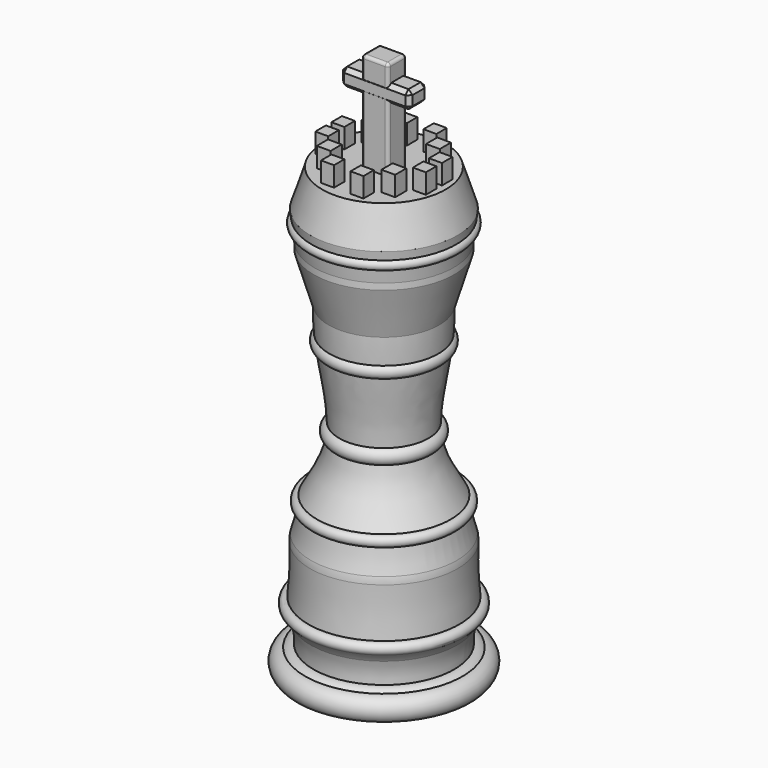
from build123d import *

# Parameters (mm, degrees)
F2_R         = 5.08
F3_W         = 3.3200064208
F3_H         = 3.3200057223
F3_W_2       = 3.5232715309
F3_H_2       = 3.5910271108
F3_W_3       = 3.3200057223
F3_H_3       = 3.3877615933
F4_DEPTH     = 5.08
F6_DEPTH     = 25.4
F7_W         = 5.9285820462
F7_H         = 4.5396015048
F8_DEPTH     = 8.89
F9_T1_DEPTH  = 1.2904933217
F9_T3_DEPTH  = 1.2904933217
F9_T5_DEPTH  = 1.2904933217
F9_T7_DEPTH  = 1.2904933217
F9_T9_DEPTH  = 1.2904933217
F9_T11_DEPTH = 1.2904933217
F9_T13_DEPTH = 1.2904933217
F9_T15_DEPTH = 1.2904933217
F9_T17_DEPTH = 9.7652613363
F9_T19_DEPTH = 11.1542418777
F9_T24_DEPTH = 23.0056598315
F9_T29_DEPTH = 23.0056598315
F9_T34_DEPTH = 23.0056598315
F9_T39_DEPTH = 23.0056598315
F9_T44_DEPTH = 23.0056598315
F9_T49_DEPTH = 23.0056598315
F9_T54_DEPTH = 23.0056598315
F9_T59_DEPTH = 23.0056598315
F9_T64_DEPTH = 23.0056598315
F9_T69_DEPTH = 23.0056598315
F9_T74_DEPTH = 23.0056598315
F9_T79_DEPTH = 23.0056598315
F10_R        = 0.762


# Not quite as in the source:
# - a fillet or chamfer that OpenCascade refuses, or shapes differently, is made with other operations: its cross-section is extruded or revolved along the edge and cut away or added


with BuildPart() as f1:
    # F0 (on Front) → F1 (revolve)
    with BuildSketch(Plane.XZ):
        with BuildLine():
            Line((0, -44.1694706678), (0, -37.9232913257))
            Line((0, -37.9232913257), (0, 63.8088807464))
            Line((0, 63.8088807464), (0, 69.7572231293))
            Line((0, 69.7572231293), (-15.8390831202, 69.7572231293))
            Line((-15.8390831202, 69.7572231293), (-18.8497721448, 60.3641234338))
            Line((-18.8497721448, 60.3641234338), (-18.5980623237, 58.2668431447))
            Line((-18.5980623237, 58.2668431447), (-18.3204592247, 55.9538165611))
            Line((-18.3204592247, 55.9538165611), (-17.942056863, 52.8009168813))
            Line((-17.942056863, 52.8009168813), (-17.9805713706, 51.2068634213))
            Line((-17.9805713706, 51.2068634213), (-14.2099214718, 38.6048460963))
            add(Edge.make_bspline(
                [(-13.9907028054, 32.0658987042), (-14.0967334303, 33.1756452858), (-14.2488688656, 35.3679737242), (-14.2418096298, 37.5414304271), (-14.2099214718, 38.6048460963)],
                knots=[0.6441859046, 0.6441859046, 0.6441859046, 0.6441859046, 0.6711541365, 0.6974927035, 0.6974927035, 0.6974927035, 0.6974927035], degree=3))
            add(Edge.make_bspline(
                [(-13.6247694985, 28.9412781618), (-13.765929725, 29.9810613532), (-13.8911317436, 31.0237597427), (-13.9907028054, 32.0658987042)],
                knots=[0.6188606226, 0.6188606226, 0.6188606226, 0.6188606226, 0.6441859046, 0.6441859046, 0.6441859046, 0.6441859046], degree=3))
            add(Edge.make_bspline(
                [(-11.4472950696, 12.1344692159), (-11.504994338, 17.2174563495), (-12.8225699529, 23.0322935701), (-13.6247694985, 28.9412781618)],
                knots=[0.4749395602, 0.4749395602, 0.4749395602, 0.4749395602, 0.6188606226, 0.6188606226, 0.6188606226, 0.6188606226], degree=3))
            add(Edge.make_bspline(
                [(-11.675667949, 8.4173418581), (-11.4991159546, 9.6023314431), (-11.4326559718, 10.8448454905), (-11.4472950696, 12.1344692159)],
                knots=[0.4384248078, 0.4384248078, 0.4384248078, 0.4384248078, 0.4749395602, 0.4749395602, 0.4749395602, 0.4749395602], degree=3))
            add(Edge.make_bspline(
                [(-17.1511071188, -4.3389676859), (-14.8148615903, -0.088300858), (-12.3768989208, 3.7107884096), (-11.675667949, 8.4173418581)],
                knots=[0.2933951502, 0.2933951502, 0.2933951502, 0.2933951502, 0.4384248078, 0.4384248078, 0.4384248078, 0.4384248078], degree=3))
            ThreePointArc((-17.1511071188, -4.3389676859), (-17.2505902332, -5.7148781332), (-17.4047115493, -7.0857439431))
            ThreePointArc((-17.4047115493, -7.0857439431), (-18.0433576285, -10.5447425672), (-19.0290799315, -13.9212632375))
            ThreePointArc((-19.0290799315, -13.9212632375), (-18.9285766864, -20.6231104547), (-19.3779931732, -27.3106273217))
            ThreePointArc((-19.3779931732, -27.3106273217), (-19.5478697821, -28.7552418846), (-19.7434488019, -30.1966017093))
            ThreePointArc((-19.7434488019, -30.1966017093), (-18.3122766997, -33.9317340327), (-18.0535539985, -37.9232913257))
            ThreePointArc((-18.0535539985, -37.9232913257), (-19.2128837803, -38.1464424542), (-20.2065406059, -38.7840066329))
            ThreePointArc((-20.2065406059, -38.7840066329), (-20.9534925411, -42.2057107785), (-18.0535539985, -44.1694706678))
            Line((-18.0535539985, -44.1694706678), (0, -44.1694706678))
        make_face()
        with BuildLine():
            Line((-22.0736673223, -44.1694706678), (-18.0535539985, -44.1694706678))
            ThreePointArc((-18.0535539985, -44.1694706678), (-20.9534925411, -42.2057107785), (-20.2065406059, -38.7840066329))
            ThreePointArc((-20.2065406059, -38.7840066329), (-22.963549203, -40.8445548127), (-22.0736673223, -44.1694706678))
        make_face()
        with BuildLine():
            Line((-18.3204592247, 55.9538165611), (-18.5980623237, 58.2668431447))
            ThreePointArc((-18.5980623237, 58.2668431447), (-19.40314177, 56.9970478477), (-18.3204592247, 55.9538165611))
        make_face()
        with BuildLine():
            ThreePointArc((-19.3779931732, -27.3106273217), (-21.0588794116, -28.5639002786), (-19.7434488019, -30.1966017093))
            ThreePointArc((-19.7434488019, -30.1966017093), (-19.5478697821, -28.7552418846), (-19.3779931732, -27.3106273217))
        make_face()
        with BuildLine():
            ThreePointArc((-18.3504191868, -6.6034462951), (-17.925820634, -6.9392158865), (-17.4047115493, -7.0857439431))
            ThreePointArc((-17.4047115493, -7.0857439431), (-17.2505902332, -5.7148781332), (-17.1511071188, -4.3389676859))
            add(Edge.make_bspline(
                [(-18.3504191868, -6.6034462951), (-17.9601567988, -5.8302207751), (-17.55716838, -5.0777732233), (-17.1511071188, -4.3389676859)],
                knots=[0.2681876432, 0.2681876432, 0.2681876432, 0.2681876432, 0.2933951502, 0.2933951502, 0.2933951502, 0.2933951502], degree=3))
        make_face()
        with BuildLine():
            add(Edge.make_bspline(
                [(-18.3504191868, -6.6034462951), (-17.9601567988, -5.8302207751), (-17.55716838, -5.0777732233), (-17.1511071188, -4.3389676859)],
                knots=[0.2681876432, 0.2681876432, 0.2681876432, 0.2681876432, 0.2933951502, 0.2933951502, 0.2933951502, 0.2933951502], degree=3))
            ThreePointArc((-17.1511071188, -4.3389676859), (-18.5181267124, -5.0647962725), (-18.3504191868, -6.6034462951))
        make_face()
        with BuildLine():
            add(Edge.make_bspline(
                [(-13.6247694985, 28.9412781618), (-13.765929725, 29.9810613532), (-13.8911317436, 31.0237597427), (-13.9907028054, 32.0658987042)],
                knots=[0.6188606226, 0.6188606226, 0.6188606226, 0.6188606226, 0.6441859046, 0.6441859046, 0.6441859046, 0.6441859046], degree=3))
            ThreePointArc((-13.9907028054, 32.0658987042), (-14.8106984904, 30.3861286262), (-13.6247694985, 28.9412781618))
        make_face()
        with BuildLine():
            ThreePointArc((-11.4472950696, 12.1344692159), (-12.8496274606, 10.355046651), (-11.675667949, 8.4173418581))
            add(Edge.make_bspline(
                [(-11.675667949, 8.4173418581), (-11.4991159546, 9.6023314431), (-11.4326559718, 10.8448454905), (-11.4472950696, 12.1344692159)],
                knots=[0.4384248078, 0.4384248078, 0.4384248078, 0.4384248078, 0.4749395602, 0.4749395602, 0.4749395602, 0.4749395602], degree=3))
        make_face()
    revolve(axis=Axis((0, 0, 12.9427947103), (0, 0, 1)))

    # F2
    f2_edges = [f1.edges().sort_by_distance(p)[0] for p in [
        (19.743449, 0, -30.196602),
        (19.02908, 0, -13.921263),
    ]]
    fillet(f2_edges, radius=F2_R)

    # F3 (on face) → F4 (join)
    with BuildSketch(Plane.XY.offset(69.7572231293)):
        with Locations((-3.7773378426, 11.6962320171)):
            Rectangle(F3_W, F3_H)
        with Locations((3.7773378426, 11.6962320171)):
            Rectangle(F3_W, F3_H)
        with Locations((-3.7773378426, -11.6962320171)):
            Rectangle(F3_W, F3_H)
        with Locations((3.7773378426, -11.6962320171)):
            Rectangle(F3_W, F3_H)
        with Locations((-8.2830600441, 7.1566319093)):
            Rectangle(F3_W_2, F3_H_2)
        with Locations((-8.2830600441, -7.1566319093)):
            Rectangle(F3_W_2, F3_H_2)
        with Locations((8.2830600441, 7.1566319093)):
            Rectangle(F3_W_2, F3_H_2)
        with Locations((8.2830600441, -7.1566319093)):
            Rectangle(F3_W_2, F3_H_2)
        with Locations((-12.5177619047, 2.583153866)):
            Rectangle(F3_W_3, F3_H_3)
        with Locations((-12.5177619047, -2.583153866)):
            Rectangle(F3_W_3, F3_H_3)
        with Locations((12.5177619047, 2.583153866)):
            Rectangle(F3_W_3, F3_H_3)
        with Locations((12.5177619047, -2.583153866)):
            Rectangle(F3_W_3, F3_H_3)
    extrude(amount=F4_DEPTH)

    # F5 (on face) → F6 (join)
    with BuildSketch(Plane.XY.offset(69.7572231293)):
        Polygon((3.4440401942, 2.9264579061), (0, 2.9264579061), (-3.4440401942, 2.9264579061), (-3.4440401942, 0), (-3.4440401942, -2.9264579061), (0, -2.9264579061), (3.4440401942, -2.9264579061), (3.4440401942, 0), align=None)
    extrude(amount=F6_DEPTH)

    # F7 (on Right) → F8 (join, symmetric)
    with BuildSketch(Plane.YZ):
        with Locations((0.0055725686, 88.3572287858)):
            Rectangle(F7_W, F7_H)
    extrude(amount=F8_DEPTH, both=True)

    # F9: chamfer of 1.016 on 12 edges, made by hand

    # F9_s2 → F9_t1 (cut)
    with BuildSketch(Plane(origin=(-33.4812493309, -33.4812493309, 33.4812493309), x_dir=(0.7071067812, -0.7071067812, 0), z_dir=(-0.5773502692, -0.5773502692, 0.5773502692))):
        Polygon((-4.9124698917, 68.7446604412), (-4.194049402, 69.9890012305), (-3.4756289123, 68.7446604412), align=None)
    extrude(amount=F9_T1_DEPTH, mode=Mode.SUBTRACT)

    # F9_s4 → F9_t3 (cut)
    with BuildSketch(Plane(origin=(25.4235698596, 25.4235698596, 25.4235698596), x_dir=(0.7071067812, -0.7071067812, 0), z_dir=(-0.5773502692, -0.5773502692, -0.5773502692))):
        Polygon((-4.9124698917, 75.5420899664), (-4.194049402, 74.2977491771), (-3.4756289123, 75.5420899664), align=None)
    extrude(amount=F9_T3_DEPTH, mode=Mode.SUBTRACT)

    # F9_s6 → F9_t5 (cut)
    with BuildSketch(Plane(origin=(-25.4235698596, 25.4235698596, 25.4235698596), x_dir=(0.7071067812, 0.7071067812, 0), z_dir=(0.5773502692, -0.5773502692, -0.5773502692))):
        Polygon((4.9124698917, 75.5420899664), (4.194049402, 74.2977491771), (3.4756289123, 75.5420899664), align=None)
    extrude(amount=F9_T5_DEPTH, mode=Mode.SUBTRACT)

    # F9_s8 → F9_t7 (cut)
    with BuildSketch(Plane(origin=(33.4812493309, -33.4812493309, 33.4812493309), x_dir=(0.7071067812, 0.7071067812, 0), z_dir=(0.5773502692, -0.5773502692, 0.5773502692))):
        Polygon((4.9124698917, 68.7446604412), (4.194049402, 69.9890012305), (3.4756289123, 68.7446604412), align=None)
    extrude(amount=F9_T7_DEPTH, mode=Mode.SUBTRACT)

    # F9_s10 → F9_t9 (cut)
    with BuildSketch(Plane(origin=(25.4198548139, -25.4198548139, 25.4198548139), x_dir=(-0.7071067812, -0.7071067812, 0), z_dir=(-0.5773502692, 0.5773502692, -0.5773502692))):
        Polygon((4.9045890895, 75.5466399497), (3.4677481102, 75.5466399497), (4.1861685998, 74.3022991603), align=None)
    extrude(amount=F9_T9_DEPTH, mode=Mode.SUBTRACT)

    # F9_s12 → F9_t11 (cut)
    with BuildSketch(Plane(origin=(-25.4198548139, -25.4198548139, 25.4198548139), x_dir=(-0.7071067812, 0.7071067812, 0), z_dir=(0.5773502692, 0.5773502692, -0.5773502692))):
        Polygon((-4.9045890895, 75.5466399497), (-3.4677481102, 75.5466399497), (-4.1861685998, 74.3022991603), align=None)
    extrude(amount=F9_T11_DEPTH, mode=Mode.SUBTRACT)

    # F9_s14 → F9_t13 (cut)
    with BuildSketch(Plane(origin=(-33.4849643766, 33.4849643766, 33.4849643766), x_dir=(-0.7071067812, -0.7071067812, 0), z_dir=(-0.5773502692, 0.5773502692, 0.5773502692))):
        Polygon((4.9045890895, 68.740110458), (3.4677481102, 68.740110458), (4.1861685998, 69.9844512473), align=None)
    extrude(amount=F9_T13_DEPTH, mode=Mode.SUBTRACT)

    # F9_s16 → F9_t15 (cut)
    with BuildSketch(Plane(origin=(33.4849643766, 33.4849643766, 33.4849643766), x_dir=(-0.7071067812, 0.7071067812, 0), z_dir=(0.5773502692, 0.5773502692, 0.5773502692))):
        Polygon((-4.9045890895, 68.740110458), (-3.4677481102, 68.740110458), (-4.1861685998, 69.9844512473), align=None)
    extrude(amount=F9_T15_DEPTH, mode=Mode.SUBTRACT)

    # F9_s18 → F9_t17 (cut)
    with BuildSketch(Plane.XY.offset(83.4745981176)):
        Polygon((-7.874, -2.9587184545), (-8.89, -1.9427184545), (-8.89, -2.9587184545), align=None)
        Polygon((7.874, -2.9587184545), (8.89, -1.9427184545), (8.89, -2.9587184545), align=None)
        Polygon((-8.89, 1.9538635917), (-7.874, 2.9698635917), (-8.89, 2.9698635917), align=None)
        Polygon((8.89, 1.9538635917), (7.874, 2.9698635917), (8.89, 2.9698635917), align=None)
    extrude(amount=F9_T17_DEPTH, mode=Mode.SUBTRACT)

    # F9_s20 → F9_t19 (cut)
    with BuildSketch(Plane.XZ.offset(-5.5826935075)):
        Polygon((7.874, 86.0874280334), (8.89, 87.1034280334), (8.89, 86.0874280334), align=None)
        Polygon((8.89, 89.6110295382), (7.874, 90.6270295382), (8.89, 90.6270295382), align=None)
        Polygon((-7.874, 86.0874280334), (-8.89, 87.1034280334), (-8.89, 86.0874280334), align=None)
        Polygon((-8.89, 89.6110295382), (-7.874, 90.6270295382), (-8.89, 90.6270295382), align=None)
    extrude(amount=F9_T19_DEPTH, mode=Mode.SUBTRACT)


with BuildPart() as f9_tool22:
    # F9_s23 → F9_t24 (new body)
    with BuildSketch(Plane.YZ.offset(-11.5028299158)):
        Polygon((-1.9427184545, 86.0874280334), (-2.9587184545, 87.1034280334), (-2.9587184545, 86.0874280334), align=None)
    extrude(amount=F9_T24_DEPTH)

    split(bisect_by=Plane.YZ.offset(-3.4440401942), keep=Keep.BOTTOM)


with BuildPart() as f1_1:
    add(f1.part)

    # F9_t21: cut F9_tool22
    add(f9_tool22.part, mode=Mode.SUBTRACT)


with BuildPart() as f9_tool27:
    # F9_s28 → F9_t29 (new body)
    with BuildSketch(Plane.YZ.offset(-11.5028299158)):
        Polygon((-1.9427184545, 86.0874280334), (-2.9587184545, 87.1034280334), (-2.9587184545, 86.0874280334), align=None)
    extrude(amount=F9_T29_DEPTH)

    split(bisect_by=Plane.XZ.offset(2.9264579061), keep=Keep.TOP)


with BuildPart() as f1_2:
    add(f1_1.part)

    # F9_t26: cut F9_tool27
    add(f9_tool27.part, mode=Mode.SUBTRACT)


with BuildPart() as f9_tool32:
    # F9_s33 → F9_t34 (new body)
    with BuildSketch(Plane.YZ.offset(-11.5028299158)):
        Polygon((-1.9427184545, 86.0874280334), (-2.9587184545, 87.1034280334), (-2.9587184545, 86.0874280334), align=None)
    extrude(amount=F9_T34_DEPTH)

    split(bisect_by=Plane.YZ.offset(3.4440401942), keep=Keep.TOP)


with BuildPart() as f1_3:
    add(f1_2.part)

    # F9_t31: cut F9_tool32
    add(f9_tool32.part, mode=Mode.SUBTRACT)


with BuildPart() as f9_tool37:
    # F9_s38 → F9_t39 (new body)
    with BuildSketch(Plane.YZ.offset(11.5028299158)):
        Polygon((-2.9587184545, 89.6110295382), (-1.9427184545, 90.6270295382), (-2.9587184545, 90.6270295382), align=None)
    extrude(amount=-F9_T39_DEPTH)

    split(bisect_by=Plane.XZ.offset(2.9264579061), keep=Keep.TOP)


with BuildPart() as f1_4:
    add(f1_3.part)

    # F9_t36: cut F9_tool37
    add(f9_tool37.part, mode=Mode.SUBTRACT)


with BuildPart() as f9_tool42:
    # F9_s43 → F9_t44 (new body)
    with BuildSketch(Plane.YZ.offset(11.5028299158)):
        Polygon((-2.9587184545, 89.6110295382), (-1.9427184545, 90.6270295382), (-2.9587184545, 90.6270295382), align=None)
    extrude(amount=-F9_T44_DEPTH)

    split(bisect_by=Plane.YZ.offset(3.4440401942), keep=Keep.TOP)


with BuildPart() as f1_5:
    add(f1_4.part)

    # F9_t41: cut F9_tool42
    add(f9_tool42.part, mode=Mode.SUBTRACT)


with BuildPart() as f9_tool47:
    # F9_s48 → F9_t49 (new body)
    with BuildSketch(Plane.YZ.offset(11.5028299158)):
        Polygon((-2.9587184545, 89.6110295382), (-1.9427184545, 90.6270295382), (-2.9587184545, 90.6270295382), align=None)
    extrude(amount=-F9_T49_DEPTH)

    split(bisect_by=Plane.YZ.offset(-3.4440401942), keep=Keep.BOTTOM)


with BuildPart() as f1_6:
    add(f1_5.part)

    # F9_t46: cut F9_tool47
    add(f9_tool47.part, mode=Mode.SUBTRACT)


with BuildPart() as f9_tool52:
    # F9_s53 → F9_t54 (new body)
    with BuildSketch(Plane.YZ.offset(-11.5028299158)):
        Polygon((1.9538635917, 86.0874280334), (2.9698635917, 87.1034280334), (2.9698635917, 86.0874280334), align=None)
    extrude(amount=F9_T54_DEPTH)

    split(bisect_by=Plane.YZ.offset(-3.4440401942), keep=Keep.BOTTOM)


with BuildPart() as f1_7:
    add(f1_6.part)

    # F9_t51: cut F9_tool52
    add(f9_tool52.part, mode=Mode.SUBTRACT)


with BuildPart() as f9_tool57:
    # F9_s58 → F9_t59 (new body)
    with BuildSketch(Plane.YZ.offset(-11.5028299158)):
        Polygon((1.9538635917, 86.0874280334), (2.9698635917, 87.1034280334), (2.9698635917, 86.0874280334), align=None)
    extrude(amount=F9_T59_DEPTH)

    split(bisect_by=Plane.XZ.offset(-2.9264579061), keep=Keep.BOTTOM)


with BuildPart() as f1_8:
    add(f1_7.part)

    # F9_t56: cut F9_tool57
    add(f9_tool57.part, mode=Mode.SUBTRACT)


with BuildPart() as f9_tool62:
    # F9_s63 → F9_t64 (new body)
    with BuildSketch(Plane.YZ.offset(-11.5028299158)):
        Polygon((1.9538635917, 86.0874280334), (2.9698635917, 87.1034280334), (2.9698635917, 86.0874280334), align=None)
    extrude(amount=F9_T64_DEPTH)

    split(bisect_by=Plane.YZ.offset(3.4440401942), keep=Keep.TOP)


with BuildPart() as f1_9:
    add(f1_8.part)

    # F9_t61: cut F9_tool62
    add(f9_tool62.part, mode=Mode.SUBTRACT)


with BuildPart() as f9_tool67:
    # F9_s68 → F9_t69 (new body)
    with BuildSketch(Plane.YZ.offset(11.5028299158)):
        Polygon((2.9698635917, 89.6110295382), (1.9538635917, 90.6270295382), (2.9698635917, 90.6270295382), align=None)
    extrude(amount=-F9_T69_DEPTH)

    split(bisect_by=Plane.XZ.offset(-2.9264579061), keep=Keep.BOTTOM)


with BuildPart() as f1_10:
    add(f1_9.part)

    # F9_t66: cut F9_tool67
    add(f9_tool67.part, mode=Mode.SUBTRACT)


with BuildPart() as f9_tool72:
    # F9_s73 → F9_t74 (new body)
    with BuildSketch(Plane.YZ.offset(11.5028299158)):
        Polygon((2.9698635917, 89.6110295382), (1.9538635917, 90.6270295382), (2.9698635917, 90.6270295382), align=None)
    extrude(amount=-F9_T74_DEPTH)

    split(bisect_by=Plane.YZ.offset(3.4440401942), keep=Keep.TOP)


with BuildPart() as f1_11:
    add(f1_10.part)

    # F9_t71: cut F9_tool72
    add(f9_tool72.part, mode=Mode.SUBTRACT)


with BuildPart() as f9_tool77:
    # F9_s78 → F9_t79 (new body)
    with BuildSketch(Plane.YZ.offset(11.5028299158)):
        Polygon((2.9698635917, 89.6110295382), (1.9538635917, 90.6270295382), (2.9698635917, 90.6270295382), align=None)
    extrude(amount=-F9_T79_DEPTH)

    split(bisect_by=Plane.YZ.offset(-3.4440401942), keep=Keep.BOTTOM)


with BuildPart() as f1_12:
    add(f1_11.part)

    # F9_t76: cut F9_tool77
    add(f9_tool77.part, mode=Mode.SUBTRACT)

    # F10
    f10_edges = [f1_12.edges().sort_by_distance(p)[0] for p in [
        (-3.44404, 2.926458, 78.408623),
        (-3.44404, -2.926458, 78.414195),
        (3.44404, 2.926458, 78.408623),
        (3.44404, -2.926458, 78.414195),
        (3.44404, -2.926458, 92.400257),
        (-3.44404, -2.926458, 92.400257),
        (3.44404, 2.926458, 92.405829),
        (-3.44404, 2.926458, 92.405829),
        (0, 2.926458, 95.157223),
        (3.44404, 0, 95.157223),
        (0, -2.926458, 95.157223),
        (-3.44404, 0, 95.157223),
    ]]
    fillet(f10_edges, radius=F10_R)


solid = f1_12.part
